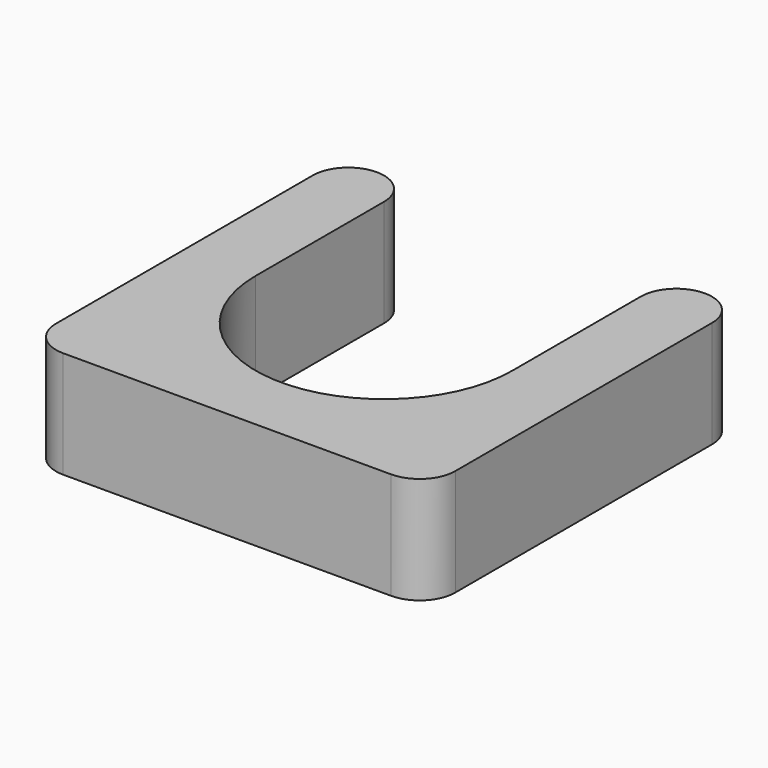
from build123d import *

# Parameters (mm, degrees)
F1_DEPTH = 25
F2_R     = 4.99999
F3_DEPTH = 15
F4_DEPTH = 10


# Not quite as in the source:
# - a fillet or chamfer is up to 0.001 mm smaller than in the source, because OpenCascade refuses the exact size


with BuildPart() as f1:
    # F0 (on Top) → F1 (new body)
    with BuildSketch(Plane.XY):
        with BuildLine():
            Line((-28, -27.5), (28, -27.5))
            Line((28, -27.5), (28, 27.5))
            Line((28, 27.5), (18, 27.5))
            Line((18, 27.5), (18, 0))
            ThreePointArc((18, 0), (0, -18), (-18, 0))
            Line((-18, 0), (-18, 27.5))
            Line((-18, 27.5), (-28, 27.5))
            Line((-28, 27.5), (-28, -27.5))
        make_face()
    extrude(amount=F1_DEPTH)

    # F2 (radius 5 in the source; OpenCascade refuses exactly that, so slightly less here)
    f2_edges = [f1.edges().sort_by_distance(p)[0] for p in [
        (18, 27.5, 12.5),
        (-18, 27.5, 12.5),
        (28, 27.5, 12.5),
        (-28, 27.5, 12.5),
        (-28, -27.5, 12.5),
        (28, -27.5, 12.5),
    ]]
    fillet(f2_edges, radius=F2_R)

    # F3 (add): a face of the model
    f3_faces = [f1.faces().sort_by_distance(p)[0] for p in [
        (0, -26.7150796219, 25),
    ]]
    extrude(f3_faces, amount=-F3_DEPTH)

    # F4 (cut): a face of the model
    f4_faces = [f1.faces().sort_by_distance(p)[0] for p in [
        (0, -26.7150796219, 25),
    ]]
    extrude(f4_faces, amount=-F4_DEPTH, mode=Mode.SUBTRACT)


solid = f1.part
